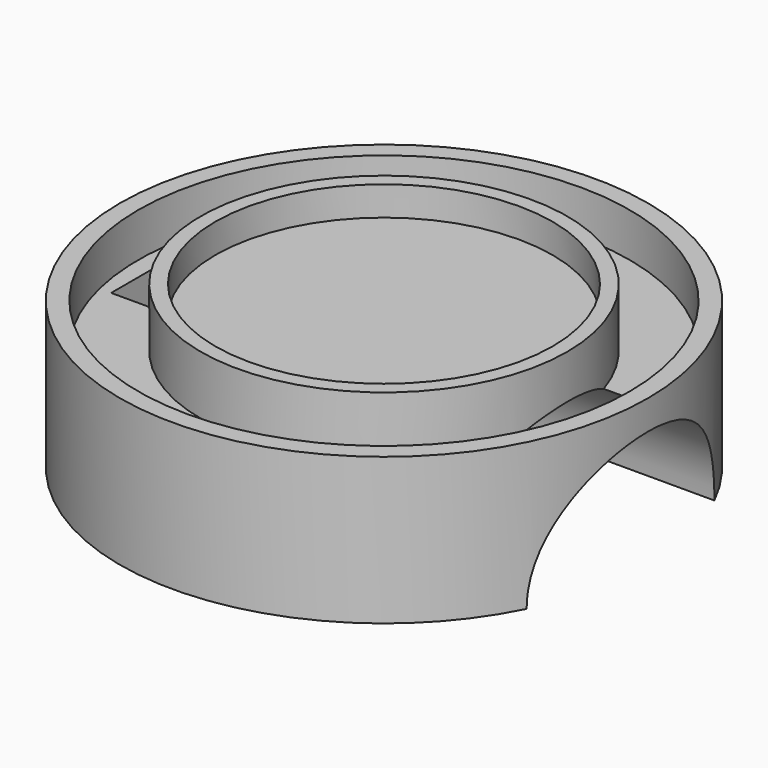
from build123d import *

# Parameters (mm, degrees)
F0_R      = 18
F0_R_2    = 16.75
F0_R_3    = 12.5
F0_R_4    = 11.5
F1_DEPTH  = 10
F2_R      = 16.75
F3_DEPTH  = 3
F4_R      = 12.5
F5_DEPTH  = 4
F6_R      = 11.5
F7_DEPTH  = 2
F9_R      = 8
F10_DEPTH = 33.5


# Not quite as in the source:
# - the program builds the solid bodies; features that only make, move or delete a surface that nothing else refers to are left out


with BuildPart() as f1:
    # F0 (on Top) → F1 (new body)
    with BuildSketch(Plane.XY):
        Circle(F0_R)
        Circle(F0_R_2, mode=Mode.SUBTRACT)
        Circle(F0_R_2)
        Circle(F0_R_3, mode=Mode.SUBTRACT)
        Circle(F0_R_3)
        Circle(F0_R_4, mode=Mode.SUBTRACT)
        Circle(F0_R_4)
    extrude(amount=F1_DEPTH)

    # F2 (on face) → F3 (cut)
    with BuildSketch(Plane.XY.offset(10)):
        Circle(F2_R)
    extrude(amount=-F3_DEPTH, mode=Mode.SUBTRACT)

    # F4 (on face) → F5 (join)
    with BuildSketch(Plane.XY.offset(7)):
        Circle(F4_R)
    extrude(amount=F5_DEPTH)

    # F6 (on face) → F7 (cut)
    with BuildSketch(Plane.XY.offset(11)):
        Circle(F6_R)
    extrude(amount=-F7_DEPTH, mode=Mode.SUBTRACT)

    # F9 (on offset) → F10 (cut)
    with BuildSketch(Plane.YZ.offset(18)):
        Circle(F9_R)
    extrude(amount=-F10_DEPTH, mode=Mode.SUBTRACT)


solid = f1.part
